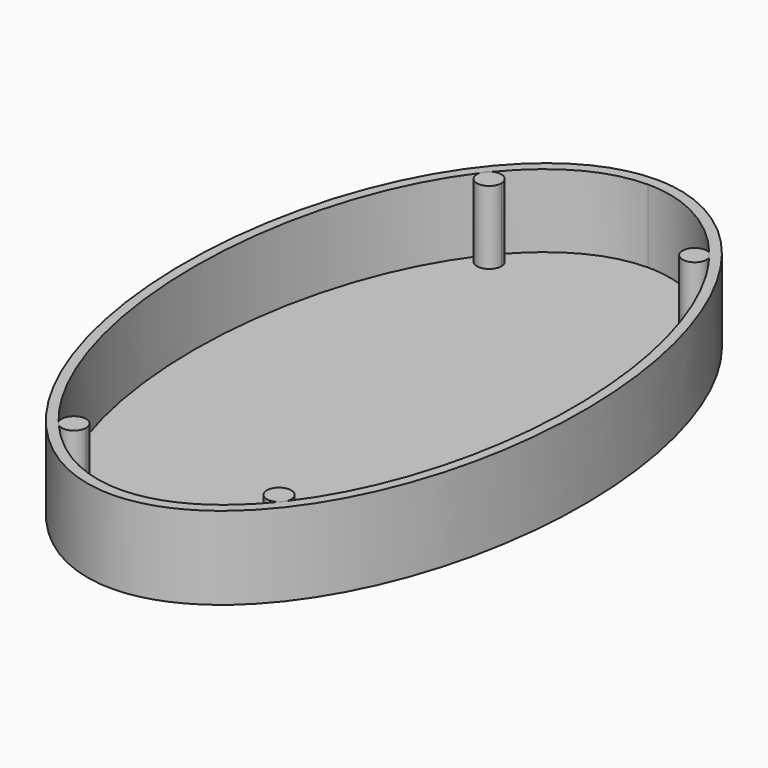
from build123d import *

# Parameters (mm, degrees)
F1_DEPTH  = 17
F3_DEPTH  = 15
F5_DEPTH  = 15
F7_DEPTH  = 15
F9_DEPTH  = 15
F11_DEPTH = 15


with BuildPart() as f1:
    # F0 (on Top) → F1 (new body)
    with BuildSketch(Plane.XY):
        with BuildLine():
            add(Edge.make_bspline(
                [(-6.2171048485, 73.2565789297), (-77.2311879588, 73.2565789297), (-41.7241464036, -31.7434210703), (-6.2171048485, -136.7434210703), (29.2899367067, -31.7434210703), (64.7969782618, 73.2565789297), (-6.2171048485, 73.2565789297)],
                knots=[0, 0, 0, 2.0943951024, 2.0943951024, 4.1887902048, 4.1887902048, 6.2831853072, 6.2831853072, 6.2831853072], degree=2, weights=[1, 0.5, 1, 0.5, 1, 0.5, 1]))
        make_face()
    extrude(amount=F1_DEPTH)

    # F2 (on face) → F3 (cut)
    with BuildSketch(Plane.XY.offset(17)):
        with BuildLine():
            add(Edge.make_bspline(
                [(-6.2171048485, 71.0526332259), (-73.7670863437, 71.0526332259), (-39.9920955961, -30.6414482184), (-6.2171048485, -132.3355296627), (27.5578858991, -30.6414482184), (61.3328766467, 71.0526332259), (-6.2171048485, 71.0526332259)],
                knots=[0, 0, 0, 2.0943951024, 2.0943951024, 4.1887902048, 4.1887902048, 6.2831853072, 6.2831853072, 6.2831853072], degree=2, weights=[1, 0.5, 1, 0.5, 1, 0.5, 1]))
        make_face()
    extrude(amount=-F3_DEPTH, mode=Mode.SUBTRACT)

    # F4 (on face) → F5 (join)
    with BuildSketch(Plane.XY.offset(2)):
        with BuildLine():
            ThreePointArc((-29.7756858862, 57.2855702673), (-27.6492449133, 54.2060390081), (-24.8481921157, 56.6878462554))
            ThreePointArc((-24.8481921157, 56.6878462554), (-26.0432758657, 58.8202612198), (-28.48594698, 58.9139446065))
            add(Edge.make_bspline(
                [(-28.48594698, 58.9139446065), (-29.1403899926, 58.1226714215), (-29.7756858862, 57.2855702673)],
                knots=[0.6420928407, 0.6420928407, 0.6420928407, 0.6808401148, 0.6808401148, 0.6808401148], degree=2, weights=[0.7874125542, 0.783834135, 0.7805979828]))
        make_face()
        with BuildLine():
            add(Edge.make_bspline(
                [(-28.48594698, 58.9139446065), (-29.1403899926, 58.1226714215), (-29.7756858862, 57.2855702673)],
                knots=[0.6420928407, 0.6420928407, 0.6420928407, 0.6808401148, 0.6808401148, 0.6808401148], degree=2, weights=[0.7874125542, 0.783834135, 0.7805979828]))
            ThreePointArc((-28.48594698, 58.9139446065), (-29.3079498058, 58.2400542943), (-29.7756858862, 57.2855702673))
        make_face()
    extrude(amount=F5_DEPTH)

    # F6 (on face) → F7 (join)
    with BuildSketch(Plane.XY.offset(2)):
        with BuildLine():
            ThreePointArc((16.1916939477, 58.7439345546), (12.7793422864, 55.3266057789), (17.4437982507, 56.577657488))
            ThreePointArc((17.4437982507, 56.577657488), (17.4180855063, 56.9352921855), (17.3414761892, 57.2855702673))
            add(Edge.make_bspline(
                [(17.3414761892, 57.2855702673), (16.7742405528, 58.0329914466), (16.1916939477, 58.7439345546)],
                knots=[5.6023451924, 5.6023451924, 5.6023451924, 5.6369260508, 5.6369260508, 5.6369260508], degree=2, weights=[0.7805979828, 0.7834861581, 0.7866469513]))
        make_face()
    extrude(amount=F7_DEPTH)

    # F8 (on face) → F9 (join)
    with BuildSketch(Plane.XY.offset(2)):
        with BuildLine():
            ThreePointArc((-27.8172974331, -53.191482885), (-25.1847662143, -53.4621797963), (-23.7840667271, -51.2168427654))
            ThreePointArc((-23.7840667271, -51.2168427654), (-26.8945171213, -48.792518052), (-28.48594698, -52.4007867471))
            add(Edge.make_bspline(
                [(-28.48594698, -52.4007867471), (-28.1539802485, -52.8021606908), (-27.8172974331, -53.191482885)],
                knots=[2.5728398269, 2.5728398269, 2.5728398269, 2.5934282254, 2.5934282254, 2.5934282254], degree=2, weights=[0.8237445465, 0.8210750527, 0.8185021925]))
        make_face()
    extrude(amount=F9_DEPTH)

    # F10 (on face) → F11 (join)
    with BuildSketch(Plane.XY.offset(2)):
        with BuildLine():
            ThreePointArc((17.2071260982, -50.948647347), (17.3423414514, -50.4905518475), (17.3879683871, -50.0151016807))
            ThreePointArc((17.3879683871, -50.0151016807), (12.6660564501, -48.8691927208), (16.3374825114, -52.0519887181))
            add(Edge.make_bspline(
                [(16.3374825114, -52.0519887181), (16.7766850943, -51.5107523345), (17.2071260982, -50.948647347)],
                knots=[3.7192756497, 3.7192756497, 3.7192756497, 3.746975358, 3.746975358, 3.746975358], degree=2, weights=[0.8260785, 0.8297264389, 0.8335492953]))
        make_face()
        with BuildLine():
            add(Edge.make_bspline(
                [(16.3374825114, -52.0519887181), (16.7766850943, -51.5107523345), (17.2071260982, -50.948647347)],
                knots=[3.7192756497, 3.7192756497, 3.7192756497, 3.746975358, 3.746975358, 3.746975358], degree=2, weights=[0.8260785, 0.8297264389, 0.8335492953]))
            ThreePointArc((16.3374825114, -52.0519887181), (16.8513996683, -51.5626602753), (17.2071260982, -50.948647347))
        make_face()
    extrude(amount=F11_DEPTH)


solid = f1.part
